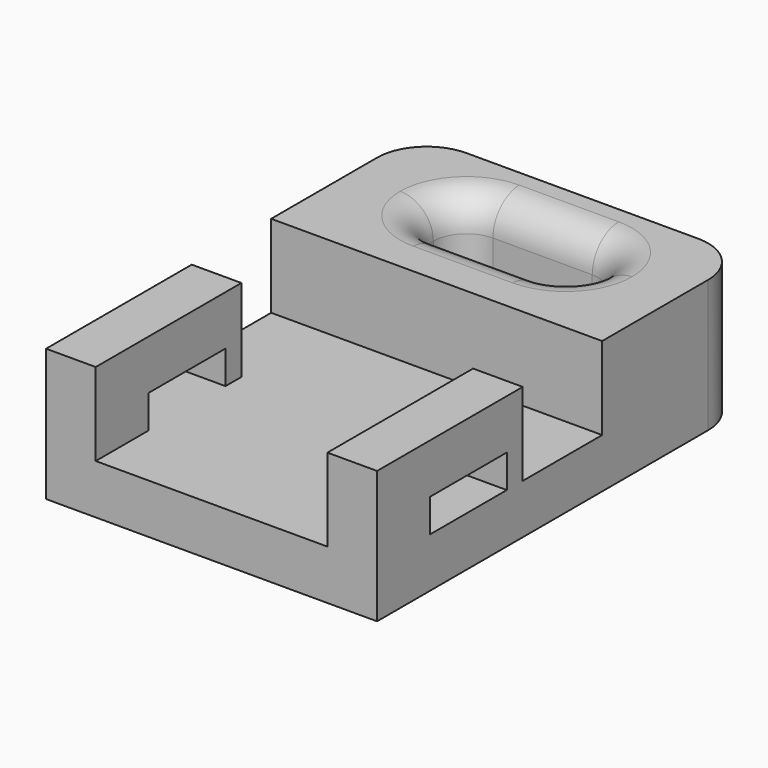
from build123d import *

# Parameters (mm, degrees)
F0_W      = 12.7
F0_H      = 15.24
F1_DEPTH  = 5.08
F2_W      = 6.35
F2_H      = 2.54
F3_DEPTH  = 25.4
F4_R      = 1.26999
F5_R      = 1.905
F6_W      = 5.715
F6_H      = 1.27
F7_DEPTH  = 25.4
F8_W      = 8.89
F8_H      = 8.255
F9_DEPTH  = 3.175
F10_W     = 1.905
F10_H     = 3.81
F11_DEPTH = 1.905
F12_DEPTH = 2.54
F13_W     = 2.5417556653
F13_H     = 1.27
F14_DEPTH = 25.4
F15_W     = 1.905
F15_H     = 0.762
F16_DEPTH = 1.27
F17_W     = 1.905
F17_H     = 0.762
F18_DEPTH = 1.27


# Not quite as in the source:
# - a fillet or chamfer is up to 0.001 mm smaller than in the source, because OpenCascade refuses the exact size


with BuildPart() as f1:
    # F0 (on Top) → F1 (new body)
    with BuildSketch(Plane.XY):
        with Locations((-20.7207803614, 14.9625845535)):
            Rectangle(F0_W, F0_H)
    extrude(amount=F1_DEPTH)

    # F2 (on face) → F3 (cut)
    with BuildSketch(Plane.XY.offset(5.08)):
        with Locations((-20.7207803614, 19.4075845535)):
            Rectangle(F2_W, F2_H)
    extrude(amount=-F3_DEPTH, mode=Mode.SUBTRACT)

    # F4 (radius 1.27 in the source; OpenCascade refuses exactly that, so slightly less here)
    f4_edges = [f1.edges().sort_by_distance(p)[0] for p in [
        (-20.72078, 18.137585, 5.08),
        (-17.54578, 19.407585, 5.08),
        (-23.89578, 19.407585, 5.08),
        (-20.72078, 20.677585, 5.08),
        (-17.54578, 19.407585, 0),
        (-20.72078, 18.137585, 0),
        (-23.89578, 19.407585, 0),
        (-20.72078, 20.677585, 0),
        (-17.54578, 18.137585, 2.54),
        (-23.89578, 18.137585, 2.54),
        (-23.89578, 20.677585, 2.54),
        (-17.54578, 20.677585, 2.54),
    ]]
    fillet(f4_edges, radius=F4_R)

    # F5
    f5_edges = [f1.edges().sort_by_distance(p)[0] for p in [
        (-27.07078, 22.582585, 2.54),
        (-14.37078, 22.582585, 2.54),
    ]]
    fillet(f5_edges, radius=F5_R)

    # F6 (on face) → F7 (cut)
    with BuildSketch(Plane.YZ.offset(-14.3707803614)):
        with Locations((12.7400845535, 2.54)):
            Rectangle(F6_W, F6_H)
    extrude(amount=-F7_DEPTH, mode=Mode.SUBTRACT)

    # F8 (on face) → F9 (cut, through all)
    with BuildSketch(Plane.XY.offset(5.08)):
        with Locations((-20.7207803614, 11.4700845535)):
            Rectangle(F8_W, F8_H)
    extrude(amount=-F9_DEPTH, mode=Mode.SUBTRACT)

    # F10 (on face) → F11 (cut, through all)
    with BuildSketch(Plane.XY.offset(5.08)):
        with Locations((-26.1182803614, 13.6925845535)):
            Rectangle(F10_W, F10_H)
        with Locations((-15.3232803614, 13.6925845535)):
            Rectangle(F10_W, F10_H)
    extrude(amount=-F11_DEPTH, mode=Mode.SUBTRACT)

    # F12 (add): a face of the model
    f12_faces = [f1.faces().sort_by_distance(p)[0] for p in [
        (-20.7207803614, 7.3425845535, 1.7991666667),
    ]]
    extrude(f12_faces, amount=F12_DEPTH)

    # F13 (on face) → F14 (cut)
    with BuildSketch(Plane.YZ.offset(-14.3707803614)):
        with Locations((8.6117067208, 2.54)):
            Rectangle(F13_W, F13_H)
    extrude(amount=-F14_DEPTH, mode=Mode.SUBTRACT)

    # F15 (on face) → F16 (join, through all)
    with BuildSketch(Plane(origin=(0, 0, 3.175), x_dir=(1, 0, 0), z_dir=(0, 0, -1))):
        with Locations((-15.3232803614, -11.4065845535)):
            Rectangle(F15_W, F15_H)
    extrude(amount=F16_DEPTH)

    # F17 (on face) → F18 (join, through all)
    with BuildSketch(Plane(origin=(0, 0, 3.175), x_dir=(1, 0, 0), z_dir=(0, 0, -1))):
        with Locations((-26.1182803614, -11.4065845535)):
            Rectangle(F17_W, F17_H)
    extrude(amount=F18_DEPTH)


solid = f1.part
